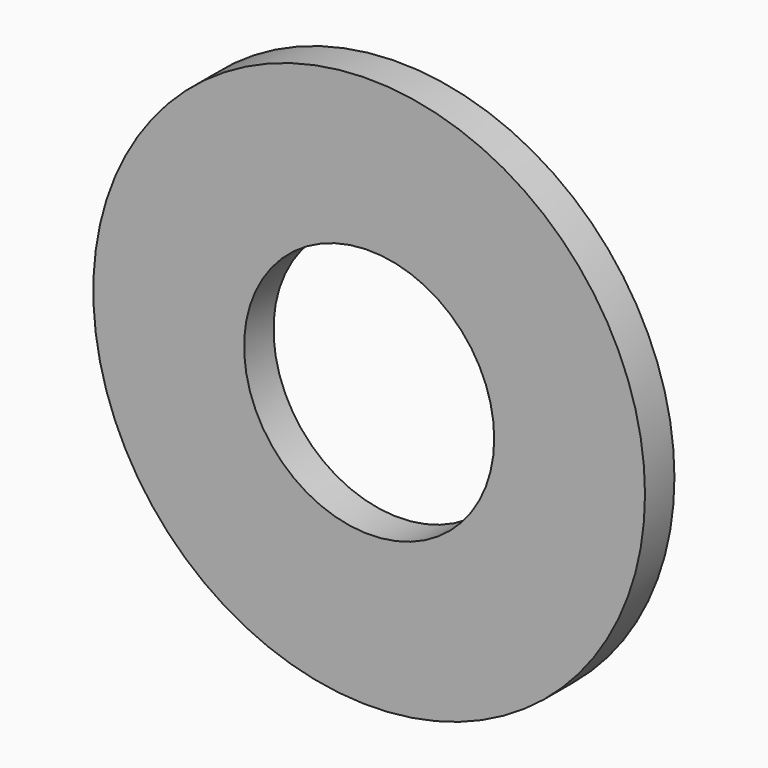
from build123d import *

# Parameters (mm, degrees)
F0_R     = 37.5
F0_R_2   = 17
F1_DEPTH = 5


# Not quite as in the source:
# - the program builds the solid bodies; features that only make, move or delete a surface that nothing else refers to are left out


with BuildPart() as f1:
    # F0 (on Front) → F1 (new body)
    with BuildSketch(Plane.XZ):
        Circle(F0_R)
        Circle(F0_R_2, mode=Mode.SUBTRACT)
    extrude(amount=F1_DEPTH)


solid = f1.part
